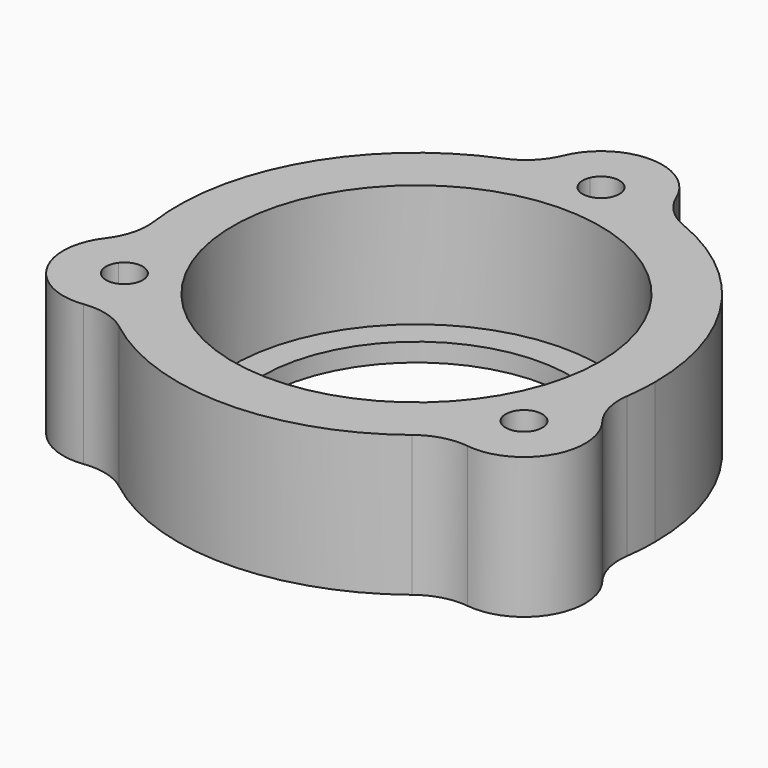
from build123d import *

# Parameters (mm, degrees)
F0_R     = 19.05
F1_DEPTH = 14.605
F0_R_2   = 16.002
F2_DEPTH = 1.905
F3_R     = 6.35


with BuildPart() as f1:
    # F0 (on Top) → F1 (new body)
    with BuildSketch(Plane.XY):
        with BuildLine():
            ThreePointArc((24.3350653445, -5.8394751301), (24.9790491411, -2.63329093), (25.194965399, 0.6297923397))
            ThreePointArc((25.194965399, 0.6297923397), (20.0585539244, 15.730247217), (6.779965399, 24.5668499075))
            ThreePointArc((6.779965399, 24.5668499075), (4.4950742876, 25.0588757184), (2.1739745412, 25.3333074158))
            ThreePointArc((2.1739745412, 25.3333074158), (2.2942832925, 24.958441266), (2.334965399, 24.5668499075))
            ThreePointArc((2.334965399, 24.5668499075), (0.0383740404, 22.702532014), (-1.3140437432, 25.3333074158))
            ThreePointArc((-1.3140437432, 25.3333074158), (-3.6351434896, 25.0588757184), (-5.920034601, 24.5668499075))
            ThreePointArc((-5.920034601, 24.5668499075), (-21.0171537257, 13.0122923397), (-23.4751345465, -5.8394751301))
            ThreePointArc((-23.4751345465, -5.8394751301), (-22.7587958424, -8.0642617829), (-21.8359107907, -10.2116089767))
            ThreePointArc((-21.8359107907, -10.2116089767), (-19.7071036642, -9.5283941084), (-18.3951345465, -11.3387364441))
            ThreePointArc((-18.3951345465, -11.3387364441), (-18.8813835693, -12.6100234553), (-20.0919016485, -13.2323214198))
            ThreePointArc((-20.0919016485, -13.2323214198), (-18.6936869538, -15.1052369163), (-17.1251345465, -16.8379977581))
            ThreePointArc((-17.1251345465, -16.8379977581), (0.429965399, -24.1352076603), (17.9850653445, -16.8379977581))
            ThreePointArc((17.9850653445, -16.8379977581), (19.5536177518, -15.1052369163), (20.9518324465, -13.2323214198))
            ThreePointArc((20.9518324465, -13.2323214198), (19.5102869503, -10.3862364441), (22.6958415887, -10.2116089767))
            ThreePointArc((22.6958415887, -10.2116089767), (23.6187266404, -8.0642617829), (24.3350653445, -5.8394751301))
        make_face()
        with Locations((0.429965399, 0.6297923397)):
            Circle(F0_R, mode=Mode.SUBTRACT)
        with BuildLine():
            ThreePointArc((-21.8359107907, -10.2116089767), (-22.7587958424, -8.0642617829), (-23.4751345465, -5.8394751301))
            ThreePointArc((-23.4751345465, -5.8394751301), (-25.7993958605, -14.5137364441), (-17.1251345465, -16.8379977581))
            ThreePointArc((-17.1251345465, -16.8379977581), (-18.6936869538, -15.1052369163), (-20.0919016485, -13.2323214198))
            ThreePointArc((-20.0919016485, -13.2323214198), (-21.9499129407, -12.2912364441), (-21.8359107907, -10.2116089767))
        make_face()
        with BuildLine():
            ThreePointArc((17.9850653445, -16.8379977581), (26.6593266585, -14.5137364441), (24.3350653445, -5.8394751301))
            ThreePointArc((24.3350653445, -5.8394751301), (23.6187266404, -8.0642617829), (22.6958415887, -10.2116089767))
            ThreePointArc((22.6958415887, -10.2116089767), (22.9704076802, -10.7457055618), (23.0650653445, -11.3387364441))
            ThreePointArc((23.0650653445, -11.3387364441), (22.4313523556, -12.7574874213), (20.9518324465, -13.2323214198))
            ThreePointArc((20.9518324465, -13.2323214198), (19.5536177518, -15.1052369163), (17.9850653445, -16.8379977581))
        make_face()
        with BuildLine():
            ThreePointArc((2.1739745412, 25.3333074158), (4.4950742876, 25.0588757184), (6.779965399, 24.5668499075))
            ThreePointArc((6.779965399, 24.5668499075), (0.429965399, 30.9168499075), (-5.920034601, 24.5668499075))
            ThreePointArc((-5.920034601, 24.5668499075), (-3.6351434896, 25.0588757184), (-1.3140437432, 25.3333074158))
            ThreePointArc((-1.3140437432, 25.3333074158), (0.429965399, 26.4718499075), (2.1739745412, 25.3333074158))
        make_face()
    extrude(amount=F1_DEPTH)

    # F0 (on Top) → F2 (join)
    with BuildSketch(Plane.XY):
        with Locations((0.429965399, 0.6297923397)):
            Circle(F0_R)
        with Locations((0.429965399, 0.6297923397)):
            Circle(F0_R_2, mode=Mode.SUBTRACT)
    extrude(amount=F2_DEPTH)

    # F3
    f3_edges = [f1.edges().sort_by_distance(p)[0] for p in [
        (17.985065, -16.837998, 7.3025),
        (-23.475135, -5.839475, 7.3025),
        (6.779965, 24.56685, 7.3025),
        (24.335065, -5.839475, 7.3025),
        (-5.920035, 24.56685, 7.3025),
        (-17.125135, -16.837998, 7.3025),
    ]]
    fillet(f3_edges, radius=F3_R)


solid = f1.part
